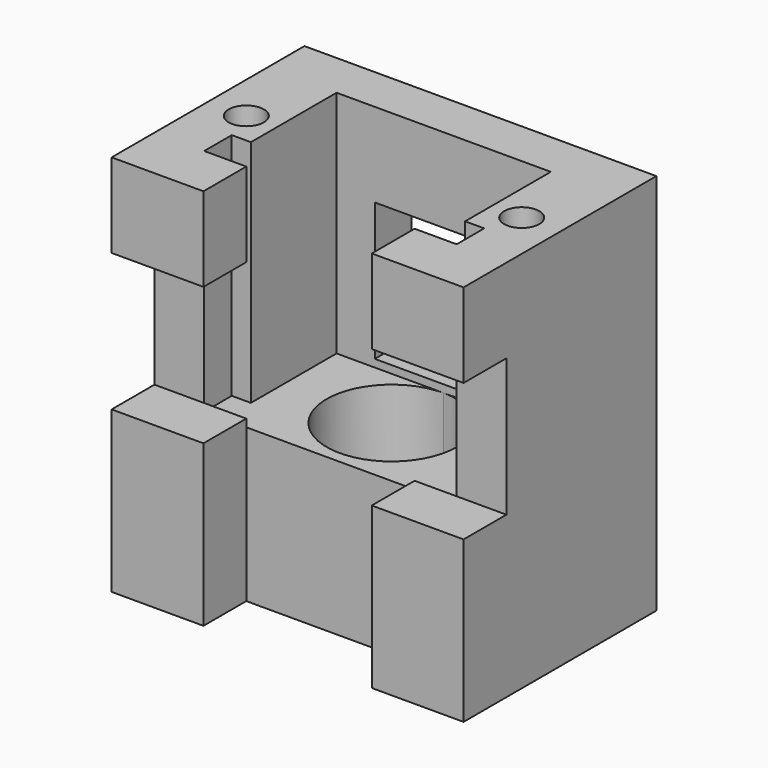
from build123d import *

# Parameters (mm, degrees)
F0_W      = 23
F0_H      = 20
F1_DEPTH  = 10
F3_DEPTH  = 15
F4_W      = 11
F4_H      = 3.5
F5_DEPTH  = 10.001
F6_DEPTH  = 3.5
F7_W      = 4.5
F7_H      = 15
F7_W_2    = 18.5
F8_DEPTH  = 3
F9_DEPTH  = 7
F10_R     = 2.5
F11_DEPTH = 10.001
F10_R_2   = 5
F12_DEPTH = 4.5
F16_R     = 1.15
F17_DEPTH = 10
F18_R     = 2.25
F19_DEPTH = 10.001
F20_DEPTH = 5
F21_DEPTH = 10.001
F22_W     = 2.5
F22_H     = 2.5
F23_DEPTH = 10.001
F24_W     = 9
F24_H     = 9
F25_DEPTH = 15.751
F26_W     = 3.5
F26_H     = 9
F27_DEPTH = 23.001


# Not quite as in the source:
# - a feature names something its author has since deleted; it is built from what else it names


with BuildPart() as f1:
    # F0 (on Top) → F1 (new body)
    with BuildSketch(Plane.XY):
        Rectangle(F0_W, F0_H)
    extrude(amount=F1_DEPTH)

    # F2 (on face) → F3 (join)
    with BuildSketch(Plane.XY.offset(10)):
        Polygon((5.5, -6.5), (5.5, -10), (11.5, -10), (11.5, -0.75), (7, -0.75), (7, -4.25), (8.25, -4.25), (8.25, -6.5), align=None)
        Polygon((-11.5, -10), (-5.5, -10), (-5.5, -6.5), (-8.25, -6.5), (-8.25, -4.25), (-7, -4.25), (-7, -0.75), (-11.5, -0.75), align=None)
    extrude(amount=F3_DEPTH)

    # F4 (on face) → F5 (cut, through all)
    with BuildSketch(Plane.XY.offset(10)):
        with Locations((0, -8.25)):
            Rectangle(F4_W, F4_H)
    extrude(amount=-F5_DEPTH, mode=Mode.SUBTRACT)

    # F6 (add): faces of the model
    f6_faces = [f1.faces().sort_by_distance(p)[0] for p in [
        (9.25, -0.75, 17.5),
        (-9.25, -0.75, 17.5),
    ]]
    extrude(f6_faces, amount=F6_DEPTH)

    # F7 (on face) → F8 (join)
    with BuildSketch(Plane(origin=(0, 2.75, 0), x_dir=(-1, 0, 0), z_dir=(0, 1, 0))):
        with Locations((-9.25, 17.5)):
            Rectangle(F7_W, F7_H)
        with Locations((2.25, 17.5)):
            Rectangle(F7_W_2, F7_H)
    extrude(amount=F8_DEPTH)

    # F9 (add): a face of the model
    f9_faces = [f1.faces().sort_by_distance(p)[0] for p in [
        (0, 10, 5),
    ]]
    extrude(f9_faces, amount=F9_DEPTH)

    # F10 (on face) → F11 (cut, through all)
    with BuildSketch(Plane.XY.offset(10)):
        with Locations((0, 11.25)):
            Circle(F10_R)
    extrude(amount=-F11_DEPTH, mode=Mode.SUBTRACT)

    # F10 (on face) → F12 (cut)
    with BuildSketch(Plane.XY.offset(10)):
        with Locations((0, 11.25)):
            Circle(F10_R_2)
        with Locations((0, 11.25)):
            Circle(F10_R, mode=Mode.SUBTRACT)
    extrude(amount=-F12_DEPTH, mode=Mode.SUBTRACT)

    # F16 (on face) → F17 (cut)
    with BuildSketch(Plane.XY.offset(25)):
        with Locations((-9, -2.125)):
            Circle(F16_R)
        with Locations((9, -2.125)):
            Circle(F16_R)
    extrude(amount=-F17_DEPTH, mode=Mode.SUBTRACT)

    # F18 (on face) → F19 (cut, through all)
    with BuildSketch(Plane.XY.offset(10)):
        with Locations((0, -1.5)):
            Circle(F18_R)
    extrude(amount=-F19_DEPTH, mode=Mode.SUBTRACT)

    # F18 (on face) → F20 (cut)
    with BuildSketch(Plane.XY.offset(10)):
        with BuildLine():
            ThreePointArc((0, 2.75), (-3.00520382, -4.50520382), (4.25, -1.5))
            ThreePointArc((4.25, -1.5), (3.00520382, 1.50520382), (0, 2.75))
        make_face()
        with Locations((0, -1.5)):
            Circle(F18_R, mode=Mode.SUBTRACT)
    extrude(amount=-F20_DEPTH, mode=Mode.SUBTRACT)

    # F21 (cut, through all): faces of the model
    f21_faces = [f1.faces().sort_by_distance(p)[0] for p in [
        (-11.2439604523, 11.375, 10),
        (-4.8585786438, 11.25, 5.5),
    ]]
    extrude(f21_faces, amount=-F21_DEPTH, mode=Mode.SUBTRACT)

    # F22 (on face) → F23 (cut, through all)
    with BuildSketch(Plane.XY.offset(10)):
        with Locations((5.75, 1.5)):
            Rectangle(F22_W, F22_H)
    extrude(amount=-F23_DEPTH, mode=Mode.SUBTRACT)

    # F24 (on face) → F25 (cut, through all)
    with BuildSketch(Plane(origin=(0, 5.75, 0), x_dir=(-1, 0, 0), z_dir=(0, 1, 0))):
        with Locations((0, 15)):
            Rectangle(F24_W, F24_H)
    extrude(amount=-F25_DEPTH, mode=Mode.SUBTRACT)

    # F26 (on face) → F27 (cut, through all)
    with BuildSketch(Plane.YZ.offset(11.5)):
        with Locations((-8.25, 15)):
            Rectangle(F26_W, F26_H)
    extrude(amount=-F27_DEPTH, mode=Mode.SUBTRACT)


solid = f1.part
